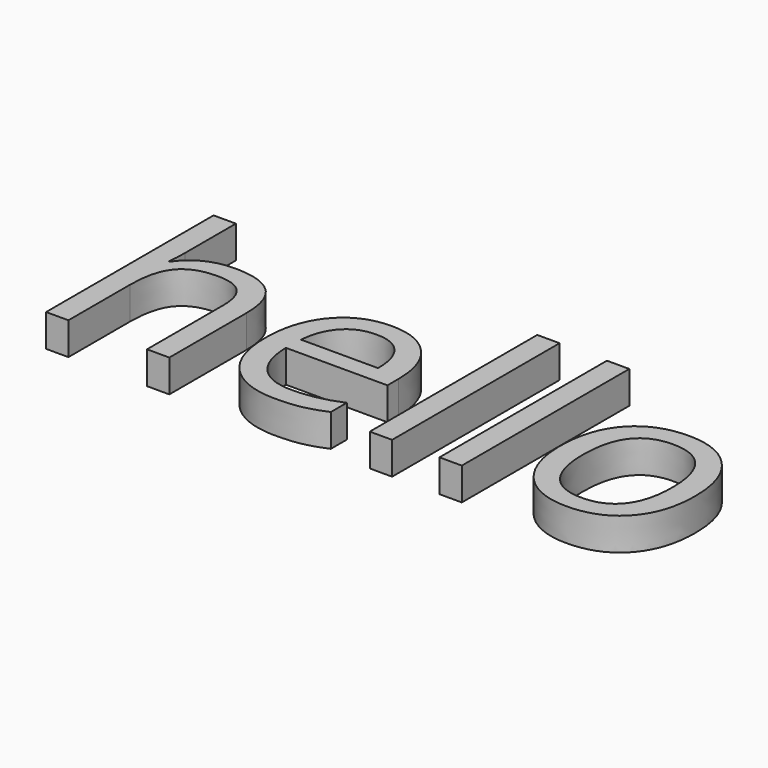
from build123d import *

# Parameters (mm, degrees)
F0_TEXT_SIZE = 576.9637309843
F1_DEPTH     = 67.9642260075


# Not quite as in the source:
# - Text() gives the source's letters only with a copy of the font that has no kerning and outlines rounded to 1/6400 em; it was checked with that copy


with BuildPart() as f1:
    # F0 (on Top) → F1 (new body)
    with BuildSketch(Plane.XY):
        with Locations((11.707178317, -415.4138863087)):
            Text('hello', F0_TEXT_SIZE, font='Open Sans', text_align=(TextAlign.LEFT, TextAlign.BOTTOM))
    extrude(amount=F1_DEPTH)


solid = f1.part
